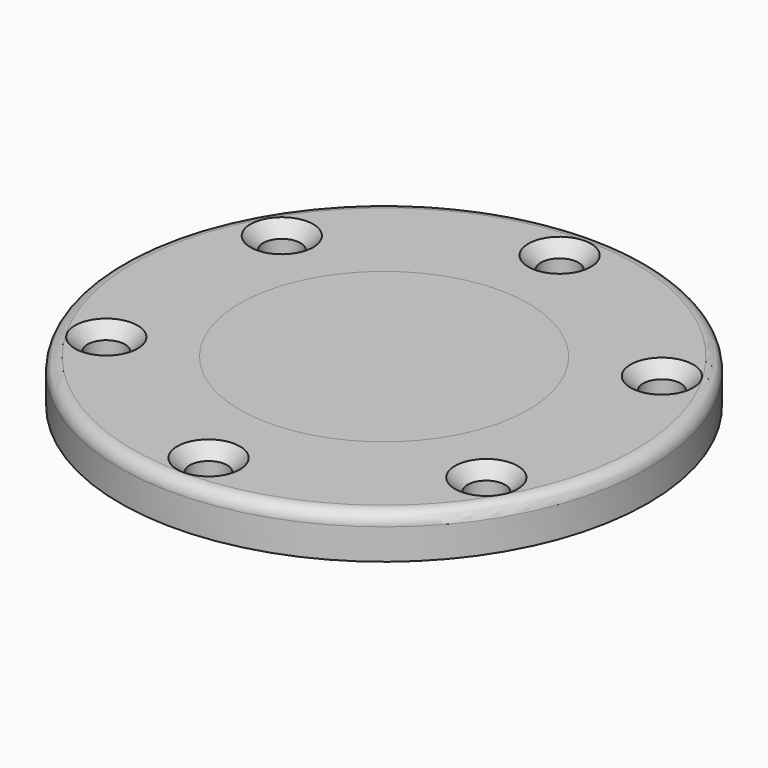
from build123d import *

# Parameters (mm, degrees)
F0_R                     = 30.6
F1_DEPTH                 = 5.7
F2_R                     = 23
F3_DEPTH                 = 1.2
F4_R                     = 2.75
F5_R                     = 42.1
F5_R_2                   = 3
F6_DEPTH                 = 6.9
F8_R                     = 5
F9_DEPTH                 = 25
DRAFT_F9_DRAFTED_ANGLE   = 45
DRAFT_F9_2_DRAFTED_ANGLE = 45
DRAFT_F9_3_DRAFTED_ANGLE = 45
DRAFT_F9_4_DRAFTED_ANGLE = 45
DRAFT_F9_5_DRAFTED_ANGLE = 45
DRAFT_F9_6_DRAFTED_ANGLE = 45
F10_R                    = 2


# Not quite as in the source:
# - an extrude with a draft is written as a straight extrude whose walls are then drafted


with BuildPart() as f1:
    # F0 (on Top) → F1 (new body)
    with BuildSketch(Plane.XY):
        Circle(F0_R)
    extrude(amount=F1_DEPTH)

    # F2 (on face) → F3 (join)
    with BuildSketch(Plane.XY.offset(5.7)):
        Circle(F2_R)
    extrude(amount=F3_DEPTH)

    # F4
    f4_edges = [f1.edges().sort_by_distance(p)[0] for p in [
        (-30.6, 0, 5.7),
    ]]
    fillet(f4_edges, radius=F4_R)


with BuildPart() as f6:
    # F5 (on Top) → F6 (new body, through all)
    with BuildSketch(Plane.XY):
        Circle(F5_R)
        with Locations((-30.3108891325, -17.5)):
            Circle(F5_R_2, mode=Mode.SUBTRACT)
        with Locations((0, -35)):
            Circle(F5_R_2, mode=Mode.SUBTRACT)
        with Locations((30.3108891325, -17.5)):
            Circle(F5_R_2, mode=Mode.SUBTRACT)
        with Locations((-30.3108891325, 17.5)):
            Circle(F5_R_2, mode=Mode.SUBTRACT)
        with Locations((30.3108891325, 17.5)):
            Circle(F5_R_2, mode=Mode.SUBTRACT)
        with Locations((0, 35)):
            Circle(F5_R_2, mode=Mode.SUBTRACT)
    extrude(amount=F6_DEPTH)

    # F7: cut F1
    add(f1.part, mode=Mode.SUBTRACT)


with BuildPart() as f9_drafted:
    # F8 (on face) → F9 (new body)
    with BuildSketch(Plane.XY.offset(6.9)):
        with Locations((-30.3108891325, -17.5)):
            Circle(F8_R)
    extrude(amount=-F9_DEPTH)

    # draft_F9_drafted
    draft_f9_drafted_walls = [f9_drafted.faces().sort_by_distance(p)[0] for p in [
        (-35.3108891325, -17.5, -9.7666666667),
    ]]
    draft(draft_f9_drafted_walls, neutral_plane=Plane(origin=(0, 0, 6.9), x_dir=(1, 0, 0), z_dir=(0, 0, -1)), angle=DRAFT_F9_DRAFTED_ANGLE)


with BuildPart() as f6_1:
    add(f6.part)

    # join_F9_drafted: cut F9_drafted
    add(f9_drafted.part, mode=Mode.SUBTRACT)


with BuildPart() as f9_2_drafted:
    # F8 (on face) → F9, piece 2 (new body)
    with BuildSketch(Plane.XY.offset(6.9)):
        with Locations((0, -35)):
            Circle(F8_R)
    extrude(amount=-F9_DEPTH)

    # draft_F9_2_drafted
    draft_f9_2_drafted_walls = [f9_2_drafted.faces().sort_by_distance(p)[0] for p in [
        (-5, -35, -9.7666666667),
    ]]
    draft(draft_f9_2_drafted_walls, neutral_plane=Plane(origin=(0, 0, 6.9), x_dir=(1, 0, 0), z_dir=(0, 0, -1)), angle=DRAFT_F9_2_DRAFTED_ANGLE)


with BuildPart() as f6_2:
    add(f6_1.part)

    # join_F9_2_drafted: cut F9_2_drafted
    add(f9_2_drafted.part, mode=Mode.SUBTRACT)


with BuildPart() as f9_3_drafted:
    # F8 (on face) → F9, piece 3 (new body)
    with BuildSketch(Plane.XY.offset(6.9)):
        with Locations((30.3108891325, -17.5)):
            Circle(F8_R)
    extrude(amount=-F9_DEPTH)

    # draft_F9_3_drafted
    draft_f9_3_drafted_walls = [f9_3_drafted.faces().sort_by_distance(p)[0] for p in [
        (25.3108891325, -17.5, -9.7666666667),
    ]]
    draft(draft_f9_3_drafted_walls, neutral_plane=Plane(origin=(0, 0, 6.9), x_dir=(1, 0, 0), z_dir=(0, 0, -1)), angle=DRAFT_F9_3_DRAFTED_ANGLE)


with BuildPart() as f6_3:
    add(f6_2.part)

    # join_F9_3_drafted: cut F9_3_drafted
    add(f9_3_drafted.part, mode=Mode.SUBTRACT)


with BuildPart() as f9_4_drafted:
    # F8 (on face) → F9, piece 4 (new body)
    with BuildSketch(Plane.XY.offset(6.9)):
        with Locations((30.3108891325, 17.5)):
            Circle(F8_R)
    extrude(amount=-F9_DEPTH)

    # draft_F9_4_drafted
    draft_f9_4_drafted_walls = [f9_4_drafted.faces().sort_by_distance(p)[0] for p in [
        (25.3108891325, 17.5, -9.7666666667),
    ]]
    draft(draft_f9_4_drafted_walls, neutral_plane=Plane(origin=(0, 0, 6.9), x_dir=(1, 0, 0), z_dir=(0, 0, -1)), angle=DRAFT_F9_4_DRAFTED_ANGLE)


with BuildPart() as f6_4:
    add(f6_3.part)

    # join_F9_4_drafted: cut F9_4_drafted
    add(f9_4_drafted.part, mode=Mode.SUBTRACT)


with BuildPart() as f9_5_drafted:
    # F8 (on face) → F9, piece 5 (new body)
    with BuildSketch(Plane.XY.offset(6.9)):
        with Locations((0, 35)):
            Circle(F8_R)
    extrude(amount=-F9_DEPTH)

    # draft_F9_5_drafted
    draft_f9_5_drafted_walls = [f9_5_drafted.faces().sort_by_distance(p)[0] for p in [
        (-5, 35, -9.7666666667),
    ]]
    draft(draft_f9_5_drafted_walls, neutral_plane=Plane(origin=(0, 0, 6.9), x_dir=(1, 0, 0), z_dir=(0, 0, -1)), angle=DRAFT_F9_5_DRAFTED_ANGLE)


with BuildPart() as f6_5:
    add(f6_4.part)

    # join_F9_5_drafted: cut F9_5_drafted
    add(f9_5_drafted.part, mode=Mode.SUBTRACT)


with BuildPart() as f9_6_drafted:
    # F8 (on face) → F9, piece 6 (new body)
    with BuildSketch(Plane.XY.offset(6.9)):
        with Locations((-30.3108891325, 17.5)):
            Circle(F8_R)
    extrude(amount=-F9_DEPTH)

    # draft_F9_6_drafted
    draft_f9_6_drafted_walls = [f9_6_drafted.faces().sort_by_distance(p)[0] for p in [
        (-35.3108891325, 17.5, -9.7666666667),
    ]]
    draft(draft_f9_6_drafted_walls, neutral_plane=Plane(origin=(0, 0, 6.9), x_dir=(1, 0, 0), z_dir=(0, 0, -1)), angle=DRAFT_F9_6_DRAFTED_ANGLE)


with BuildPart() as f6_6:
    add(f6_5.part)

    # join_F9_6_drafted: cut F9_6_drafted
    add(f9_6_drafted.part, mode=Mode.SUBTRACT)

    # F10
    f10_edges = [f6_6.edges().sort_by_distance(p)[0] for p in [
        (-42.1, 0, 6.9),
    ]]
    fillet(f10_edges, radius=F10_R)


solid = Compound([f1.part, f6_6.part])
